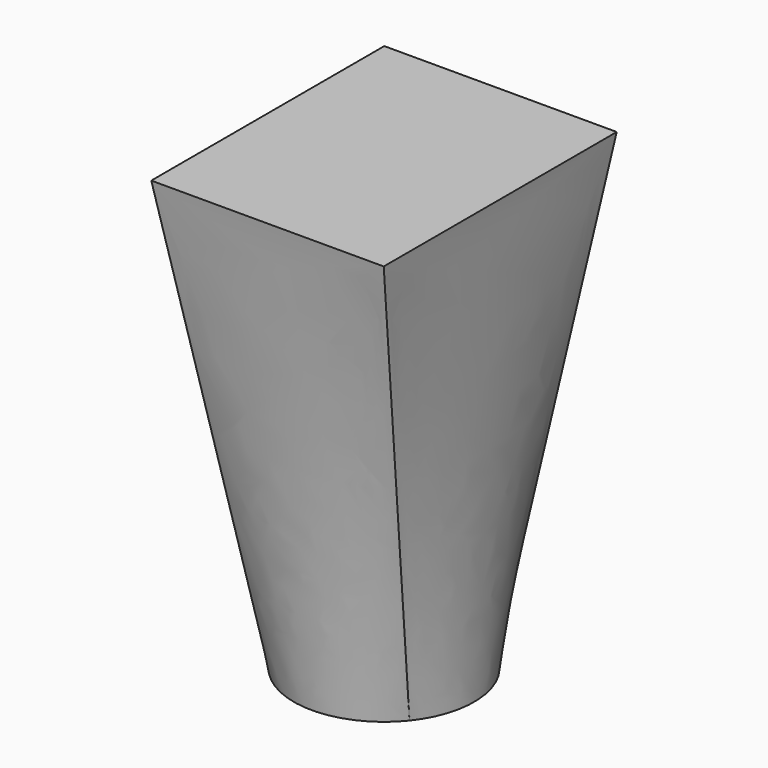
from build123d import *

# Parameters (mm, degrees)
F2_W = 51.5391305089
F2_H = 64.5755082369


# Not quite as in the source:
# - the arcs of a loft's sections are written as splines that run evenly, so that the points pair up as in the source's solid


with BuildPart() as f3:
    # F0 (on Top) → F3 section 0
    with BuildSketch(Plane.XY):
        with BuildLine():
            add(Edge.make_bspline(
                [(12.4759920731, 15.6316864667), (11.4529005863, 16.4482382384), (10.3494130561, 17.1640065946), (8.0239442184, 18.3665400162), (6.8020204126, 18.8532753465), (4.2866321741, 19.5790259612), (2.9932299393, 19.8180232999), (0.3845872594, 20.0391009186), (-0.930588682, 20.021175732), (-3.5322371281, 19.7290844658), (-4.8186453021, 19.4549256087), (-7.3133196237, 18.6608903611), (-8.5215240856, 18.1410336047), (-10.8133553474, 16.875568705), (-11.8969254774, 16.1299918528), (-13.8978398894, 14.4417284075), (-14.8151346949, 13.4990835599), (-15.6316864667, 12.4759920731)],
                knots=[0, 0, 0, 0, 0.125, 0.125, 0.25, 0.25, 0.375, 0.375, 0.5, 0.5, 0.625, 0.625, 0.75, 0.75, 0.875, 0.875, 1, 1, 1, 1], degree=3))
            add(Edge.make_bspline(
                [(-15.6316864667, 12.4759920731), (-16.4482382384, 11.4529005863), (-17.1640065946, 10.3494130561), (-18.3665400162, 8.0239442184), (-18.8532753465, 6.8020204126), (-19.5790259612, 4.2866321741), (-19.8180232999, 2.9932299393), (-20.0391009186, 0.3845872594), (-20.021175732, -0.930588682), (-19.7290844658, -3.5322371281), (-19.4549256087, -4.8186453021), (-18.6608903611, -7.3133196237), (-18.1410336047, -8.5215240856), (-16.875568705, -10.8133553474), (-16.1299918528, -11.8969254774), (-14.4417284075, -13.8978398894), (-13.4990835599, -14.8151346949), (-12.4759920731, -15.6316864667)],
                knots=[0, 0, 0, 0, 0.125, 0.125, 0.25, 0.25, 0.375, 0.375, 0.5, 0.5, 0.625, 0.625, 0.75, 0.75, 0.875, 0.875, 1, 1, 1, 1], degree=3))
            add(Edge.make_bspline(
                [(-12.4759920731, -15.6316864667), (-11.4529005863, -16.4482382384), (-10.3494130561, -17.1640065946), (-8.0239442184, -18.3665400162), (-6.8020204126, -18.8532753465), (-4.2866321741, -19.5790259612), (-2.9932299393, -19.8180232999), (-0.3845872594, -20.0391009186), (0.930588682, -20.021175732), (3.5322371281, -19.7290844658), (4.8186453021, -19.4549256087), (7.3133196237, -18.6608903611), (8.5215240856, -18.1410336047), (10.8133553474, -16.875568705), (11.8969254774, -16.1299918528), (13.8978398894, -14.4417284075), (14.8151346949, -13.4990835599), (15.6316864667, -12.4759920731)],
                knots=[0, 0, 0, 0, 0.125, 0.125, 0.25, 0.25, 0.375, 0.375, 0.5, 0.5, 0.625, 0.625, 0.75, 0.75, 0.875, 0.875, 1, 1, 1, 1], degree=3))
            add(Edge.make_bspline(
                [(15.6316864667, -12.4759920731), (16.4482382384, -11.4529005863), (17.1640065946, -10.3494130561), (18.3665400162, -8.0239442184), (18.8532753465, -6.8020204126), (19.5790259612, -4.2866321741), (19.8180232999, -2.9932299393), (20.0391009186, -0.3845872594), (20.021175732, 0.930588682), (19.7290844658, 3.5322371281), (19.4549256087, 4.8186453021), (18.6608903611, 7.3133196237), (18.1410336047, 8.5215240856), (16.875568705, 10.8133553474), (16.1299918528, 11.8969254774), (14.4417284075, 13.8978398894), (13.4990835599, 14.8151346949), (12.4759920731, 15.6316864667)],
                knots=[0, 0, 0, 0, 0.125, 0.125, 0.25, 0.25, 0.375, 0.375, 0.5, 0.5, 0.625, 0.625, 0.75, 0.75, 0.875, 0.875, 1, 1, 1, 1], degree=3))
        make_face()
    # F2 (on offset) → F3 section 1
    with BuildSketch(Plane.XY.offset(100)):
        Rectangle(F2_W, F2_H)
    loft(ruled=True)


solid = f3.part
